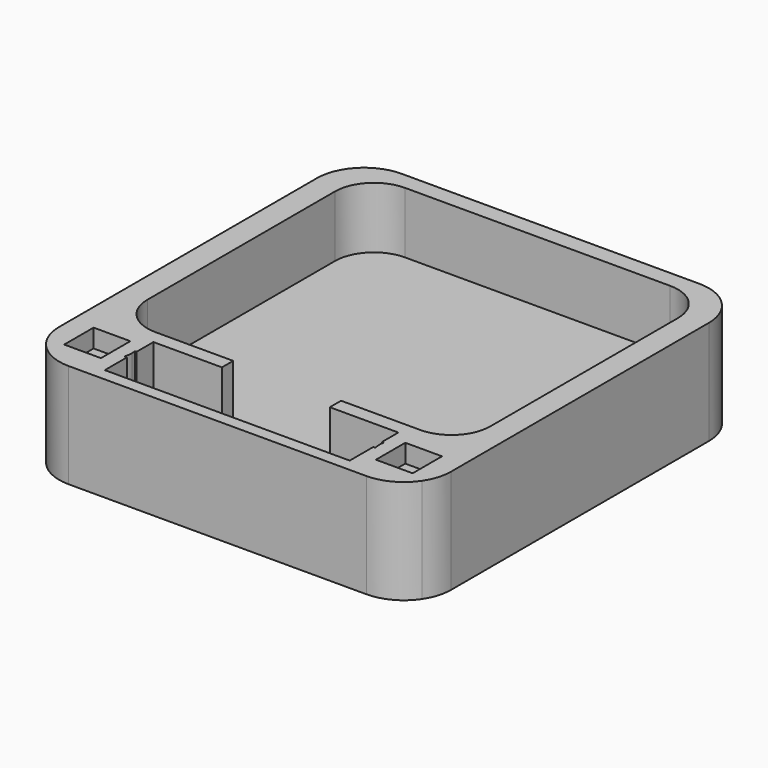
from build123d import *

# Parameters (mm, degrees)
F1_DEPTH  = 17
F2_DEPTH  = 5
F3_DEPTH  = 17
F4_DEPTH  = 3
F5_W      = 17.619991675
F5_H      = 2.2976936506
F6_DEPTH  = 10
F7_W      = 10
F7_H      = 4
F7_W_2    = 40
F7_H_2    = 5
F8_DEPTH  = 3
F9_W      = 6
F9_H      = 6
F10_DEPTH = 3


# Not quite as in the source:
# - a feature names something its author has since deleted; it is built from what else it names


with BuildPart() as f1:
    # F0 (on Top) → F1 (new body)
    with BuildSketch(Plane.XY):
        with BuildLine():
            Line((24.3022678875, 34), (-24.3022678875, 34))
            ThreePointArc((-24.3022678875, 34), (-29.745386464, 31.745386464), (-32, 26.3022678875))
            Line((-32, 26.3022678875), (-32, 15.1276998222))
            Line((-32, 15.1276998222), (-30.5, 15.1276998222))
            Line((-30.5, 15.1276998222), (-30.5, 21.3020170704))
            Line((-30.5, 21.3020170704), (30.5, 21.3020170704))
            Line((30.5, 21.3020170704), (30.5, 14.2477769405))
            Line((30.5, 14.2477769405), (32, 14.2477769405))
            Line((32, 14.2477769405), (32, 26.3022678875))
            ThreePointArc((32, 26.3022678875), (29.745386464, 31.745386464), (24.3022678875, 34))
        make_face()
        with BuildLine():
            Line((-30.5, 15.1276998222), (-32, 15.1276998222))
            Line((-32, 15.1276998222), (-32, -26.3022678875))
            ThreePointArc((-32, -26.3022678875), (-29.745386464, -31.745386464), (-24.3022678875, -34))
            Line((-24.3022678875, -34), (0, -34))
            Line((0, -34), (0, -32))
            Line((0, -32), (-20, -32))
            Line((-20, -32), (-20, -27.4899639189))
            Line((-20, -27.4899639189), (-20.3994758379, -27.4899639189))
            ThreePointArc((-20.3994758379, -27.4899639189), (-30.2031719041, -25.7844938681), (-20.255592559, -25.5261339915))
            Line((-20.255592559, -25.5261339915), (-20, -25.5261339915))
            Line((-20, -25.5261339915), (-20, -22.0704134554))
            Line((-20, -22.0704134554), (-4.1499226354, -22.0704134554))
            Line((-4.1499226354, -22.0704134554), (-4.1499226354, -14.6979829296))
            Line((-4.1499226354, -14.6979829296), (-30.5, -14.6979829296))
            Line((-30.5, -14.6979829296), (-30.5, 15.1276998222))
        make_face()
        with BuildLine():
            Line((32, -26.3022678875), (32, 14.2477769405))
            Line((32, 14.2477769405), (30.5, 14.2477769405))
            Line((30.5, 14.2477769405), (30.5, -14.6979829296))
            Line((30.5, -14.6979829296), (4.1499226354, -14.6979829296))
            Line((4.1499226354, -14.6979829296), (4.1499226354, -22.0704134554))
            Line((4.1499226354, -22.0704134554), (20, -22.0704134554))
            Line((20, -22.0704134554), (20, -25.4029799253))
            Line((20, -25.4029799253), (20.2726339823, -25.4029799253))
            ThreePointArc((20.2726339823, -25.4029799253), (25.5910239568, -21.1638916046), (30.2165381279, -26.1498479185))
            ThreePointArc((30.2165381279, -26.1498479185), (25.7296627026, -31.1234485429), (20.3218568596, -27.1706786007))
            Line((20.3218568596, -27.1706786007), (20, -27.1706786007))
            Line((20, -27.1706786007), (20, -32))
            Line((20, -32), (0, -32))
            Line((0, -32), (0, -34))
            Line((0, -34), (24.3022678875, -34))
            ThreePointArc((24.3022678875, -34), (27.9138443036, -33.100178998), (30.6810753302, -30.6110838832))
            ThreePointArc((30.6810753302, -30.6110838832), (31.6628871063, -28.555346757), (32, -26.3022678875))
        make_face()
        Polygon((-30.5, 21.3020170704), (-30.5, 15.1276998222), (-30.5, -14.6979829296), (-4.1499226354, -14.6979829296), (4.1499226354, -14.6979829296), (30.5, -14.6979829296), (30.5, 14.2477769405), (30.5, 21.3020170704), align=None)
        Polygon((4.1499226354, -14.6979829296), (-4.1499226354, -14.6979829296), (-4.1499226354, -22.0704134554), (0, -22.0704134554), (4.1499226354, -22.0704134554), align=None)
        with BuildLine():
            ThreePointArc((20.2726339823, -25.4029799253), (20.2184754644, -26.2890226707), (20.3218568596, -27.1706786007))
            ThreePointArc((20.3218568596, -27.1706786007), (25.7296627026, -31.1234485429), (30.2165381279, -26.1498479185))
            ThreePointArc((30.2165381279, -26.1498479185), (25.5910239568, -21.1638916046), (20.2726339823, -25.4029799253))
        make_face()
    extrude(amount=F1_DEPTH)

    # F0 (on Top) → F2 (cut)
    with BuildSketch(Plane.XY):
        Polygon((-30.5, 21.3020170704), (-30.5, 15.1276998222), (-30.5, -14.6979829296), (-4.1499226354, -14.6979829296), (4.1499226354, -14.6979829296), (30.5, -14.6979829296), (30.5, 14.2477769405), (30.5, 21.3020170704), align=None)
        Polygon((4.1499226354, -14.6979829296), (-4.1499226354, -14.6979829296), (-4.1499226354, -22.0704134554), (0, -22.0704134554), (4.1499226354, -22.0704134554), align=None)
    extrude(amount=F2_DEPTH, mode=Mode.SUBTRACT)

    # F0 (on Top) → F3 (join)
    with BuildSketch(Plane.XY):
        with BuildLine():
            ThreePointArc((-20.255592559, -25.5261339915), (-30.2031719041, -25.7844938681), (-20.3994758379, -27.4899639189))
            ThreePointArc((-20.3994758379, -27.4899639189), (-20.2624836545, -26.8261202565), (-20.2165381279, -26.1498479185))
            ThreePointArc((-20.2165381279, -26.1498479185), (-20.2263112871, -25.8373801956), (-20.255592559, -25.5261339915))
        make_face()
    extrude(amount=F3_DEPTH)

    # F0 (on Top) → F4 (cut)
    with BuildSketch(Plane.XY):
        with BuildLine():
            ThreePointArc((20.2726339823, -25.4029799253), (20.2184754644, -26.2890226707), (20.3218568596, -27.1706786007))
            ThreePointArc((20.3218568596, -27.1706786007), (25.7296627026, -31.1234485429), (30.2165381279, -26.1498479185))
            ThreePointArc((30.2165381279, -26.1498479185), (25.5910239568, -21.1638916046), (20.2726339823, -25.4029799253))
        make_face()
        with BuildLine():
            ThreePointArc((-20.255592559, -25.5261339915), (-30.2031719041, -25.7844938681), (-20.3994758379, -27.4899639189))
            ThreePointArc((-20.3994758379, -27.4899639189), (-20.2624836545, -26.8261202565), (-20.2165381279, -26.1498479185))
            ThreePointArc((-20.2165381279, -26.1498479185), (-20.2263112871, -25.8373801956), (-20.255592559, -25.5261339915))
        make_face()
    extrude(amount=F4_DEPTH, mode=Mode.SUBTRACT)

    # F5 (on face) → F6 (cut)
    with BuildSketch(Plane.XY.offset(17)):
        with BuildLine():
            Line((21.7456496224, 31.2272801952), (-21.5543503776, 31.2272801952))
            ThreePointArc((-21.5543503776, 31.2272801952), (-26.0444784382, 29.3674082557), (-27.9043503776, 24.8772801952))
            Line((-27.9043503776, 24.8772801952), (-27.9043503776, -13.4227198048))
            ThreePointArc((-27.9043503776, -13.4227198048), (-26.0444784382, -17.9128478653), (-21.5543503776, -19.7727198048))
            Line((-21.5543503776, -19.7727198048), (-8.8099958375, -19.7727198048))
            Line((-8.8099958375, -19.7727198048), (8.8099958375, -19.7727198048))
            Line((8.8099958375, -19.7727198048), (21.7456496224, -19.7727198048))
            ThreePointArc((21.7456496224, -19.7727198048), (26.2357776829, -17.9128478653), (28.0956496224, -13.4227198048))
            Line((28.0956496224, -13.4227198048), (28.0956496224, 24.8772801952))
            ThreePointArc((28.0956496224, 24.8772801952), (26.2357776829, 29.3674082557), (21.7456496224, 31.2272801952))
        make_face()
        with Locations((0, -20.9215666301)):
            Rectangle(F5_W, F5_H)
    extrude(amount=-F6_DEPTH, mode=Mode.SUBTRACT)

    # F7 (on face) → F8 (cut)
    with BuildSketch(Plane.XY):
        with Locations((-14.1091264039, -18.375430584)):
            Rectangle(F7_W, F7_H)
        with Locations((14.1091264039, -18.375430584)):
            Rectangle(F7_W, F7_H)
        with Locations((-1.1501409858, 27.3545110226)):
            Rectangle(F7_W_2, F7_H_2)
    extrude(amount=F8_DEPTH, mode=Mode.SUBTRACT)

    # F9 (on face) → F10 (cut)
    with BuildSketch(Plane.XY.offset(17)):
        with Locations((25.4528271034, -26.7212770808)):
            Rectangle(F9_W, F9_H)
        with Locations((-25.4528271034, -26.7212770808)):
            Rectangle(F9_W, F9_H)
    extrude(amount=-F10_DEPTH, mode=Mode.SUBTRACT)


solid = f1.part
